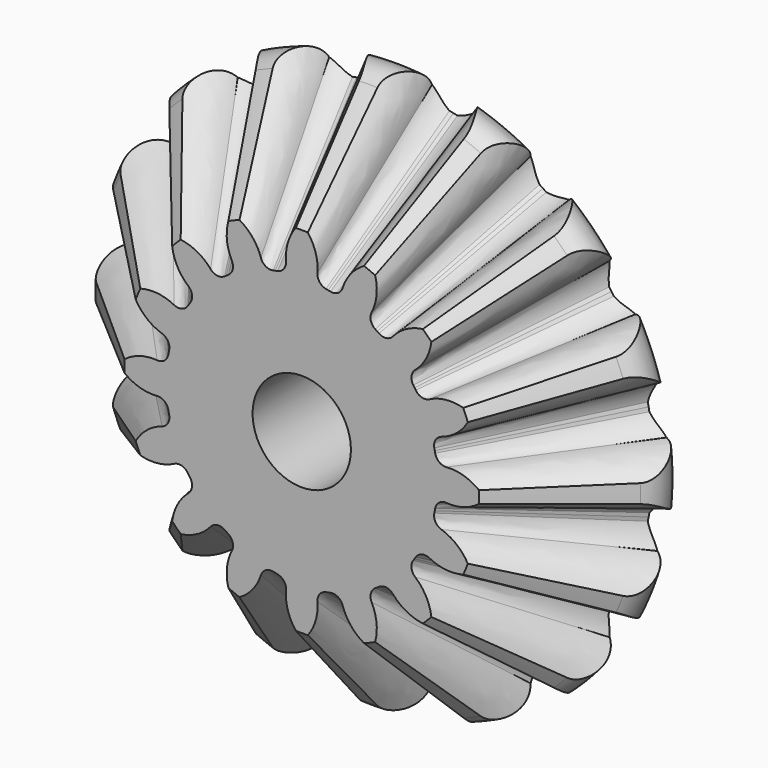
from build123d import *

# Parameters (mm, degrees)
F2_R             = 13
F3_DEPTH         = 0.05
F5_DEPTH         = 0.05
F7_DEPTH         = 0.05
F24_COPIES_COUNT = 16
F25_T2_ANGLE     = 65.4289068252
F25_T4_ANGLE     = 65.4289068252
F25_T6_ANGLE     = 65.4289068252
F25_T8_ANGLE     = 65.4289068252
F25_T10_ANGLE    = 65.4289068252
F25_T12_ANGLE    = 65.4289068252
F25_T14_ANGLE    = 65.4289068252
F25_T16_ANGLE    = 65.4289068252
F25_T18_ANGLE    = 65.4289068252
F25_T20_ANGLE    = 65.4289068252
F25_T22_ANGLE    = 65.4289068252
F25_T24_ANGLE    = 65.4289068252
F25_T26_ANGLE    = 65.4289068252
F25_T28_ANGLE    = 65.4289068252
F25_T30_ANGLE    = 65.4289068252
F25_T32_ANGLE    = 65.4289068252
F26_R            = 4.7625
F27_DEPTH        = 12.7510001
F28_R            = 38.1
F29_DEPTH        = 0.254


# Not quite as in the source:
# - a fillet or chamfer that OpenCascade refuses, or shapes differently, is made with other operations: its cross-section is extruded or revolved along the edge and cut away or added
# - a pattern or mirror of a feature is missing from the dataset's text; its kind, count and spacing are read off the source's solid


with BuildPart() as f3:
    # F2 (on Front) → F3 (new body, symmetric)
    with BuildSketch(Plane.XZ):
        Circle(F2_R)
    extrude(amount=F3_DEPTH, both=True)



with BuildPart() as f5:
    # F4 (on Front) → F5 (new body, symmetric)
    with BuildSketch(Plane.XZ):
        with BuildLine():
            ThreePointArc((-1.3290517168, 12.9318839128), (0, 13), (1.3290517168, 12.9318839128))
            ThreePointArc((1.3290517168, 12.9318839128), (1.4474573198, 15.0526353047), (0.5771423279, 16.9902003147))
            ThreePointArc((0.5771423279, 16.9902003147), (0, 17), (-0.5771423279, 16.9902003147))
            ThreePointArc((-0.5771423279, 16.9902003147), (-1.4474573198, 15.0526353047), (-1.3290517168, 12.9318839128))
        make_face()
    extrude(amount=F5_DEPTH, both=True)


with BuildPart() as f3_1:
    add(f3.part)

    add(f5.part)  # F7 merges F5
    # F6 (on Front) → F7 (join, symmetric)
    with BuildSketch(Plane.XZ):
        with BuildLine():
            ThreePointArc((2.3243525127, 12.790519356), (1.7091695194, 13.1664607203), (1.5066827152, 13.8584008323))
            Line((1.5066827152, 13.8584008323), (-1.5066827152, 13.8584008323))
            ThreePointArc((-1.5066827152, 13.8584008323), (-1.7091695194, 13.1664607203), (-2.3243525127, 12.790519356))
            ThreePointArc((-2.3243525127, 12.790519356), (0, 13), (2.3243525127, 12.790519356))
        make_face()
    extrude(amount=F7_DEPTH, both=True)

    # F22 (on offset) → F24 section 0
    with BuildSketch(Plane.XZ.offset(-12.7)):
        with BuildLine():
            ThreePointArc((2.78827014, 25.646385161), (2.3652860838, 28.6627474273), (1.0672485374, 31.4181884738))
            ThreePointArc((1.0672485374, 31.4181884738), (0, 31.43631), (-1.0672485374, 31.4181884738))
            ThreePointArc((-1.0672485374, 31.4181884738), (-2.3652860838, 28.6627474273), (-2.78827014, 25.646385161))
            ThreePointArc((-2.78827014, 25.646385161), (-3.4025350819, 24.5496706606), (-4.3016398601, 23.6711977172))
            ThreePointArc((-4.3016398601, 23.6711977172), (-4.497801929, 23.6347093204), (-4.6936546465, 23.596595367))
            Line((-4.6936546465, 23.596595367), (0, 0))
            Line((0, 0), (4.6936546465, 23.596595367))
            ThreePointArc((4.6936546465, 23.596595367), (4.497801929, 23.6347093204), (4.3016398601, 23.6711977172))
            ThreePointArc((4.3016398601, 23.6711977172), (3.4025350819, 24.5496706606), (2.78827014, 25.646385161))
        make_face()
    # F23 (on face) → F24 section 1
    with BuildSketch(Plane(origin=(0, 0.05, 0), x_dir=(-1, 0, 0), z_dir=(0, 1, 0))):
        with BuildLine():
            ThreePointArc((-0.5771423279, 16.9902003147), (-1.3370779818, 15.5119077839), (-1.5066827152, 13.8584008323))
            ThreePointArc((-1.5066827152, 13.8584008323), (-1.7091695194, 13.1664607203), (-2.3243525127, 12.790519356))
            ThreePointArc((-2.3243525127, 12.790519356), (-2.4303469271, 12.7708031781), (-2.5361741862, 12.7502086452))
            Line((-2.5361741862, 12.7502086452), (0, 0))
            Line((0, 0), (2.5361741862, 12.7502086452))
            ThreePointArc((2.5361741862, 12.7502086452), (2.4303469271, 12.7708031781), (2.3243525127, 12.790519356))
            ThreePointArc((2.3243525127, 12.790519356), (1.7091695194, 13.1664607203), (1.5066827152, 13.8584008323))
            ThreePointArc((1.5066827152, 13.8584008323), (1.3370779818, 15.5119077839), (0.5771423279, 16.9902003147))
            ThreePointArc((0.5771423279, 16.9902003147), (0, 17), (-0.5771423279, 16.9902003147))
        make_face()
    f24 = loft()

    # F24_copies: F24 ×16 about axis
    f24_copies_axis = Axis((0, 0, 0), (0, 1, 0))
    for i in range(1, F24_COPIES_COUNT):
        add(f24.rotate(f24_copies_axis, i * 360 / F24_COPIES_COUNT))

    # F25: fillet of radius 2.54 on 16 edges, made by hand

    # F25_s1 → F25_t2 (revolve, cut)
    with BuildSketch(Plane(origin=(0, 0, 0), x_dir=(0, 1, 0), z_dir=(0.8413744743, 0, -0.5404525825))):
        with BuildLine():
            ThreePointArc((8.2496511104, 26.3575261124), (11.0542353774, 27.0609401953), (12.7, 24.6835586336))
            Line((12.7, 24.6835586336), (12.7, 31.43631))
            Line((12.7, 31.43631), (8.2496511104, 26.3575261124))
        make_face()
    revolve(axis=Axis((0, 12.7, 0), (0, -1, 0)), revolution_arc=F25_T2_ANGLE, mode=Mode.SUBTRACT)

    # F25_s3 → F25_t4 (revolve, cut)
    with BuildSketch(Plane(origin=(0, 0, 0), x_dir=(0, 1, 0), z_dir=(0.5705064067, 0, -0.821293151))):
        with BuildLine():
            ThreePointArc((12.7, 24.6835586336), (11.0542353774, 27.0609401953), (8.2496511104, 26.3575261124))
            Line((8.2496511104, 26.3575261124), (12.7, 31.43631))
            Line((12.7, 31.43631), (12.7, 24.6835586336))
        make_face()
    revolve(axis=Axis((0, 12.7, 0), (0, -1, 0)), revolution_arc=F25_T4_ANGLE, mode=Mode.SUBTRACT)

    # F25_s5 → F25_t6 (revolve, cut)
    with BuildSketch(Plane(origin=(0, 0, 0), x_dir=(0, 1, 0), z_dir=(0.2127839103, 0, -0.9770992823))):
        with BuildLine():
            ThreePointArc((12.7, 24.6835586336), (11.0542353774, 27.0609401953), (8.2496511104, 26.3575261124))
            Line((8.2496511104, 26.3575261124), (12.7, 31.43631))
            Line((12.7, 31.43631), (12.7, 24.6835586336))
        make_face()
    revolve(axis=Axis((0, 12.7, 0), (0, -1, 0)), revolution_arc=F25_T6_ANGLE, mode=Mode.SUBTRACT)

    # F25_s7 → F25_t8 (revolve, cut)
    with BuildSketch(Plane(origin=(0, 0, 0), x_dir=(0, 1, 0), z_dir=(-0.1773330075, 0, -0.9841509053))):
        with BuildLine():
            ThreePointArc((12.7, 24.6835586336), (11.0542353774, 27.0609401953), (8.2496511104, 26.3575261124))
            Line((8.2496511104, 26.3575261124), (12.7, 31.43631))
            Line((12.7, 31.43631), (12.7, 24.6835586336))
        make_face()
    revolve(axis=Axis((0, 12.7, 0), (0, -1, 0)), revolution_arc=F25_T8_ANGLE, mode=Mode.SUBTRACT)

    # F25_s9 → F25_t10 (revolve, cut)
    with BuildSketch(Plane(origin=(0, 0, 0), x_dir=(0, 1, 0), z_dir=(-0.5404525825, 0, -0.8413744743))):
        with BuildLine():
            ThreePointArc((12.7, 24.6835586336), (11.0542353774, 27.0609401953), (8.2496511104, 26.3575261124))
            Line((8.2496511104, 26.3575261124), (12.7, 31.43631))
            Line((12.7, 31.43631), (12.7, 24.6835586336))
        make_face()
    revolve(axis=Axis((0, 12.7, 0), (0, -1, 0)), revolution_arc=F25_T10_ANGLE, mode=Mode.SUBTRACT)

    # F25_s11 → F25_t12 (revolve, cut)
    with BuildSketch(Plane(origin=(0, 0, 0), x_dir=(0, 1, 0), z_dir=(-0.821293151, 0, -0.5705064067))):
        with BuildLine():
            ThreePointArc((12.7, 24.6835586336), (11.0542353774, 27.0609401953), (8.2496511104, 26.3575261124))
            Line((8.2496511104, 26.3575261124), (12.7, 31.43631))
            Line((12.7, 31.43631), (12.7, 24.6835586336))
        make_face()
    revolve(axis=Axis((0, 12.7, 0), (0, -1, 0)), revolution_arc=F25_T12_ANGLE, mode=Mode.SUBTRACT)

    # F25_s13 → F25_t14 (revolve, cut)
    with BuildSketch(Plane(origin=(0, 0, 0), x_dir=(0, 1, 0), z_dir=(-0.9770992823, 0, -0.2127839103))):
        with BuildLine():
            ThreePointArc((12.7, 24.6835586336), (11.0542353774, 27.0609401953), (8.2496511104, 26.3575261124))
            Line((8.2496511104, 26.3575261124), (12.7, 31.43631))
            Line((12.7, 31.43631), (12.7, 24.6835586336))
        make_face()
    revolve(axis=Axis((0, 12.7, 0), (0, -1, 0)), revolution_arc=F25_T14_ANGLE, mode=Mode.SUBTRACT)

    # F25_s15 → F25_t16 (revolve, cut)
    with BuildSketch(Plane(origin=(0, 0, 0), x_dir=(0, 1, 0), z_dir=(-0.9841509053, 0, 0.1773330075))):
        with BuildLine():
            ThreePointArc((12.7, 24.6835586336), (11.0542353774, 27.0609401953), (8.2496511104, 26.3575261124))
            Line((8.2496511104, 26.3575261124), (12.7, 31.43631))
            Line((12.7, 31.43631), (12.7, 24.6835586336))
        make_face()
    revolve(axis=Axis((0, 12.7, 0), (0, -1, 0)), revolution_arc=F25_T16_ANGLE, mode=Mode.SUBTRACT)

    # F25_s17 → F25_t18 (revolve, cut)
    with BuildSketch(Plane(origin=(0, 0, 0), x_dir=(0, 1, 0), z_dir=(-0.8413744743, 0, 0.5404525825))):
        with BuildLine():
            ThreePointArc((12.7, 24.6835586336), (11.0542353774, 27.0609401953), (8.2496511104, 26.3575261124))
            Line((8.2496511104, 26.3575261124), (12.7, 31.43631))
            Line((12.7, 31.43631), (12.7, 24.6835586336))
        make_face()
    revolve(axis=Axis((0, 12.7, 0), (0, -1, 0)), revolution_arc=F25_T18_ANGLE, mode=Mode.SUBTRACT)

    # F25_s19 → F25_t20 (revolve, cut)
    with BuildSketch(Plane(origin=(0, 0, 0), x_dir=(0, 1, 0), z_dir=(-0.5705064067, 0, 0.821293151))):
        with BuildLine():
            ThreePointArc((12.7, 24.6835586336), (11.0542353774, 27.0609401953), (8.2496511104, 26.3575261124))
            Line((8.2496511104, 26.3575261124), (12.7, 31.43631))
            Line((12.7, 31.43631), (12.7, 24.6835586336))
        make_face()
    revolve(axis=Axis((0, 12.7, 0), (0, -1, 0)), revolution_arc=F25_T20_ANGLE, mode=Mode.SUBTRACT)

    # F25_s21 → F25_t22 (revolve, cut)
    with BuildSketch(Plane(origin=(0, 0, 0), x_dir=(0, 1, 0), z_dir=(-0.2127839103, 0, 0.9770992823))):
        with BuildLine():
            ThreePointArc((12.7, 24.6835586336), (11.0542353774, 27.0609401953), (8.2496511104, 26.3575261124))
            Line((8.2496511104, 26.3575261124), (12.7, 31.43631))
            Line((12.7, 31.43631), (12.7, 24.6835586336))
        make_face()
    revolve(axis=Axis((0, 12.7, 0), (0, -1, 0)), revolution_arc=F25_T22_ANGLE, mode=Mode.SUBTRACT)

    # F25_s23 → F25_t24 (revolve, cut)
    with BuildSketch(Plane(origin=(0, 0, 0), x_dir=(0, 1, 0), z_dir=(0.1773330075, 0, 0.9841509053))):
        with BuildLine():
            ThreePointArc((12.7, 24.6835586336), (11.0542353774, 27.0609401953), (8.2496511104, 26.3575261124))
            Line((8.2496511104, 26.3575261124), (12.7, 31.43631))
            Line((12.7, 31.43631), (12.7, 24.6835586336))
        make_face()
    revolve(axis=Axis((0, 12.7, 0), (0, -1, 0)), revolution_arc=F25_T24_ANGLE, mode=Mode.SUBTRACT)

    # F25_s25 → F25_t26 (revolve, cut)
    with BuildSketch(Plane(origin=(0, 0, 0), x_dir=(0, 1, 0), z_dir=(0.5404525825, 0, 0.8413744743))):
        with BuildLine():
            ThreePointArc((12.7, 24.6835586336), (11.0542353774, 27.0609401953), (8.2496511104, 26.3575261124))
            Line((8.2496511104, 26.3575261124), (12.7, 31.43631))
            Line((12.7, 31.43631), (12.7, 24.6835586336))
        make_face()
    revolve(axis=Axis((0, 12.7, 0), (0, -1, 0)), revolution_arc=F25_T26_ANGLE, mode=Mode.SUBTRACT)

    # F25_s27 → F25_t28 (revolve, cut)
    with BuildSketch(Plane(origin=(0, 0, 0), x_dir=(0, 1, 0), z_dir=(0.821293151, 0, 0.5705064067))):
        with BuildLine():
            ThreePointArc((12.7, 24.6835586336), (11.0542353774, 27.0609401953), (8.2496511104, 26.3575261124))
            Line((8.2496511104, 26.3575261124), (12.7, 31.43631))
            Line((12.7, 31.43631), (12.7, 24.6835586336))
        make_face()
    revolve(axis=Axis((0, 12.7, 0), (0, -1, 0)), revolution_arc=F25_T28_ANGLE, mode=Mode.SUBTRACT)

    # F25_s29 → F25_t30 (revolve, cut)
    with BuildSketch(Plane(origin=(0, 0, 0), x_dir=(0, 1, 0), z_dir=(0.9770992823, 0, 0.2127839103))):
        with BuildLine():
            ThreePointArc((12.7, 24.6835586336), (11.0542353774, 27.0609401953), (8.2496511104, 26.3575261124))
            Line((8.2496511104, 26.3575261124), (12.7, 31.43631))
            Line((12.7, 31.43631), (12.7, 24.6835586336))
        make_face()
    revolve(axis=Axis((0, 12.7, 0), (0, -1, 0)), revolution_arc=F25_T30_ANGLE, mode=Mode.SUBTRACT)

    # F25_s31 → F25_t32 (revolve, cut)
    with BuildSketch(Plane(origin=(0, 0, 0), x_dir=(0, 1, 0), z_dir=(0.9841509053, 0, -0.1773330075))):
        with BuildLine():
            ThreePointArc((12.7, 24.6835586336), (11.0542353774, 27.0609401953), (8.2496511104, 26.3575261124))
            Line((8.2496511104, 26.3575261124), (12.7, 31.43631))
            Line((12.7, 31.43631), (12.7, 24.6835586336))
        make_face()
    revolve(axis=Axis((0, 12.7, 0), (0, -1, 0)), revolution_arc=F25_T32_ANGLE, mode=Mode.SUBTRACT)

    # F26 (on face) → F27 (cut, through all)
    with BuildSketch(Plane.XZ.offset(0.05)):
        Circle(F26_R)
    extrude(amount=-F27_DEPTH, mode=Mode.SUBTRACT)

    # F28 (on face) → F29 (cut)
    with BuildSketch(Plane.XZ.offset(0.05)):
        Circle(F28_R)
    extrude(amount=-F29_DEPTH, mode=Mode.SUBTRACT)


solid = f3_1.part
